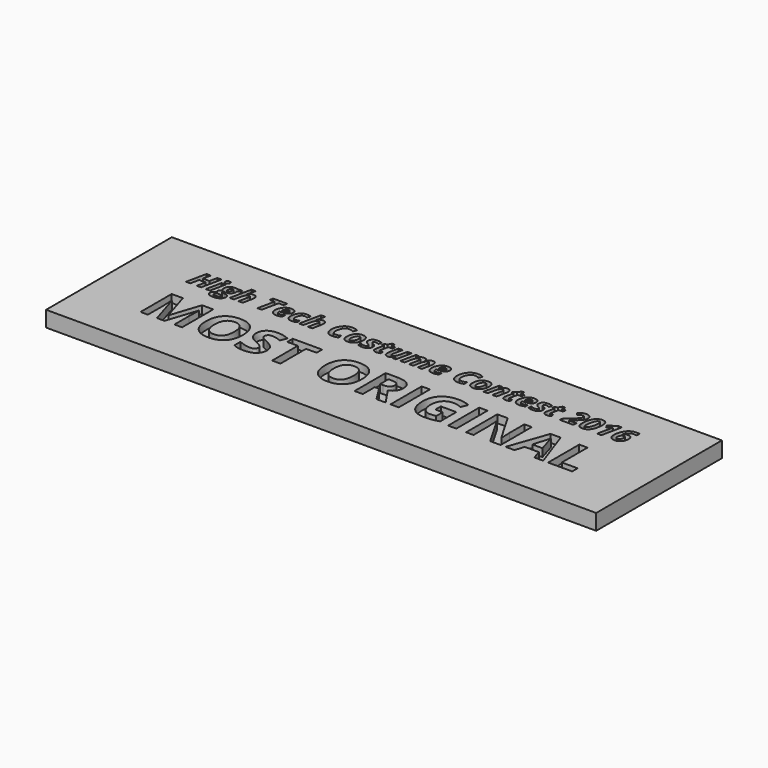
from build123d import *

# Parameters (mm, degrees)
F1_W           = 88.9
F1_H           = 25.4
F2_DEPTH       = 2.54
F0_TEXT_SIZE   = 4.6078496877
F0_TEXT_SIZE_2 = 8.8135698242
F3_DEPTH       = 1.27


# Not quite as in the source:
# - Text() gives the source's letters only with a copy of the font that has no kerning and outlines rounded to 1/6400 em; it was checked with that copy


with BuildPart() as f2:
    # F1 (on face) → F2 (new body)
    with BuildSketch(Plane.XY):
        with Locations((44.45, 12.7)):
            Rectangle(F1_W, F1_H)
    extrude(amount=-F2_DEPTH)

    # F0 (on Top) → F3 (cut)
    with BuildSketch(Plane.XY):
        with Locations((8.89, 17.0023482249)):
            Text('High Tech Costume Contest 2016', F0_TEXT_SIZE, font='Open Sans', font_style=FontStyle.BOLDITALIC, text_align=(TextAlign.LEFT, TextAlign.BOTTOM))
        with Locations((8.89, 6.9702401298)):
            Text('MOST ORIGINAL', F0_TEXT_SIZE_2, font='Open Sans', font_style=FontStyle.BOLD, text_align=(TextAlign.LEFT, TextAlign.BOTTOM))
    extrude(amount=-F3_DEPTH, mode=Mode.SUBTRACT)


solid = f2.part
